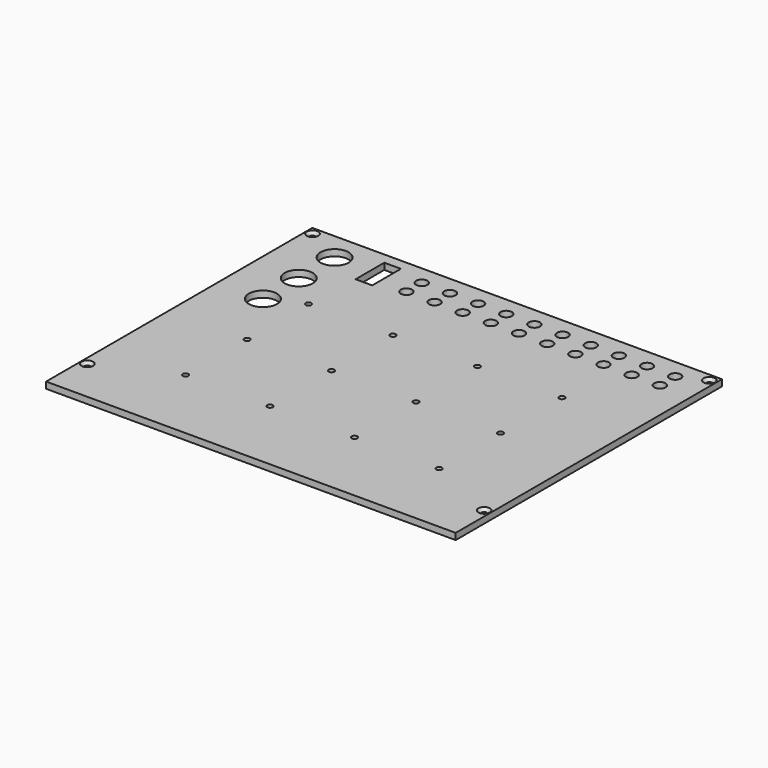
from build123d import *

# Parameters (mm, degrees)
F0_W           = 320
F0_H           = 260
F1_DEPTH       = 2.5
F3_D           = 4.4
F3_DEPTH       = 17.25
F3_CSINK_D     = 8.96
F3_CSINK_ANGLE = 90
F3_TIP         = 1.3218933619
F5_D           = 8.8
F5_DEPTH       = 17.25
F5_TIP         = 2.6437867237
F7_D           = 4.4
F7_DEPTH       = 17.25
F7_TIP         = 1.3218933619
F9_D           = 22
F9_DEPTH       = 17.25
F9_TIP         = 6.6094668093
F10_W          = 13
F10_H          = 28
F11_DEPTH      = 25


# Not quite as in the source:
# - a feature names something its author has since deleted; it is built from what else it names


with BuildPart() as f1:
    # F0 (on Top) → F1 (new body, symmetric)
    with BuildSketch(Plane.XY):
        Rectangle(F0_W, F0_H)
    extrude(amount=F1_DEPTH, both=True)

    # F3
    with Locations(Plane.XY.offset(2.5)):
        with Locations((-155, -96), (-155, 124), (155, 124), (155, -96)):
            CounterSinkHole(F3_D / 2, F3_CSINK_D / 2, depth=F3_DEPTH, counter_sink_angle=F3_CSINK_ANGLE)
            with Locations((0, 0, -(F3_DEPTH + F3_TIP / 2))):  # 118° drill point
                Cone(0, F3_D / 2, F3_TIP, mode=Mode.SUBTRACT)

    # F5
    with Locations(Plane.XY.offset(2.5)):
        with Locations((-62.5, 115), (-62.5, 100), (-40.5, 115), (-40.5, 100), (-18.5, 115), (3.5, 100), (3.5, 115), (-18.5, 100), (25.5, 100), (25.5, 115), (47.5, 115), (69.5, 115), (91.5, 115), (91.5, 100), (113.5, 100), (113.5, 115), (47.5, 100), (69.5, 100), (135.5, 115), (135.5, 100)):
            Hole(F5_D / 2, depth=F5_DEPTH)
            with Locations((0, 0, -(F5_DEPTH + F5_TIP / 2))):  # 118° drill point
                Cone(0, F5_D / 2, F5_TIP, mode=Mode.SUBTRACT)

    # F7
    with Locations(Plane.XY.offset(2.5)):
        with Locations((-99, 50), (-99, -10), (-99, -70), (-33, -70), (-33, -10), (-33, 50), (33, 50), (99, 50), (99, -10), (33, -10), (33, -70), (99, -70)):
            Hole(F7_D / 2, depth=F7_DEPTH)
            with Locations((0, 0, -(F7_DEPTH + F7_TIP / 2))):  # 118° drill point
                Cone(0, F7_D / 2, F7_TIP, mode=Mode.SUBTRACT)

    # F9
    with Locations(Plane.XY.offset(2.5)):
        with Locations((-125, 108), (-125, 73), (-125, 38)):
            Hole(F9_D / 2, depth=F9_DEPTH)
            with Locations((0, 0, -(F9_DEPTH + F9_TIP / 2))):  # 118° drill point
                Cone(0, F9_D / 2, F9_TIP, mode=Mode.SUBTRACT)

    # F10 (on face) → F11 (cut)
    with BuildSketch(Plane.XY.offset(2.5)):
        with Locations((-90.5, 107.5)):
            Rectangle(F10_W, F10_H)
    extrude(amount=-F11_DEPTH, mode=Mode.SUBTRACT)


solid = f1.part
